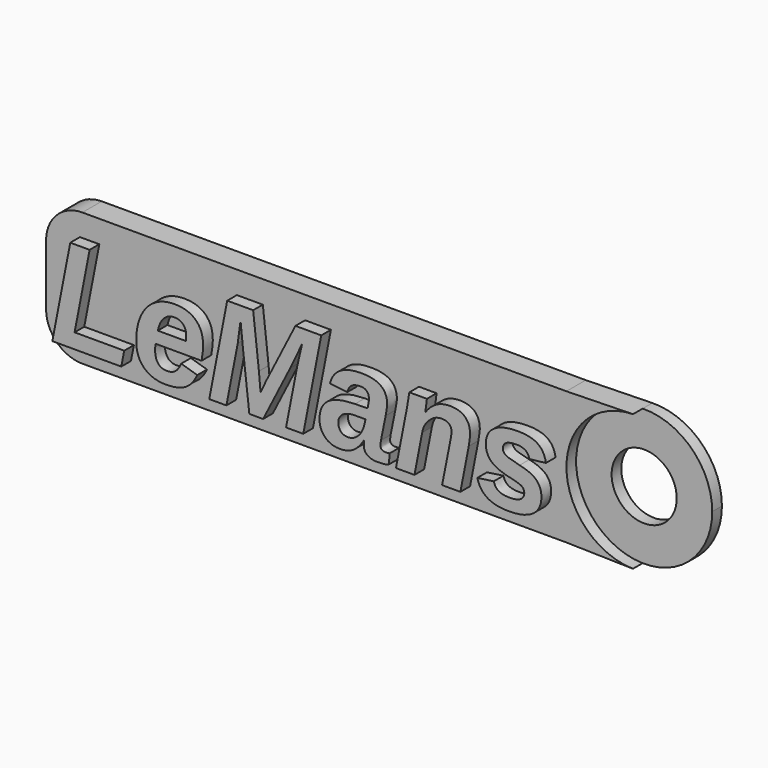
from build123d import *

# Parameters (mm, degrees)
F0_TEXT_SIZE = 11.1111111111
F1_DEPTH     = 1
F2_R         = 2.69
F3_DEPTH     = 2
F4_R         = 3
F5_R         = 5.625
F6_DEPTH     = 1


# Not quite as in the source:
# - Text() gives the source's letters only with a copy of the font that has no kerning and outlines rounded to 1/6400 em; it was checked with that copy


with BuildPart() as f1:
    # F0 (on Front) → F1 (new body)
    with BuildSketch(Plane.XZ):
        with Locations((-20.8784722222, -8)):
            Text('LeMans', F0_TEXT_SIZE, font='Arimo', font_style=FontStyle.BOLDITALIC, text_align=(TextAlign.LEFT, TextAlign.BOTTOM))
    extrude(amount=F1_DEPTH)


with BuildPart() as f3:
    # F2 (on Front) → F3 (new body)
    with BuildSketch(Plane.XZ):
        with BuildLine():
            Line((-22, -9.5), (21, -9.5))
            Line((21, -9.5), (26.4986114618, -9.6235799041))
            ThreePointArc((26.4986114618, -9.6235799041), (21, -4), (26.4986114618, 1.6235799041))
            Line((26.4986114618, 1.6235799041), (21, 1.5))
            Line((21, 1.5), (-22, 1.5))
            Line((-22, 1.5), (-22, -9.5))
        make_face()
        with BuildLine():
            ThreePointArc((26.4986114618, 1.6235799041), (21, -4), (26.4986114618, -9.6235799041))
            ThreePointArc((26.4986114618, -9.6235799041), (30.5575366796, -8.0219125132), (32.25, -4))
            ThreePointArc((32.25, -4), (30.5575366796, 0.0219125132), (26.4986114618, 1.6235799041))
        make_face()
        with Locations((26.625, -4)):
            Circle(F2_R, mode=Mode.SUBTRACT)
    extrude(amount=-F3_DEPTH)

    # F4
    f4_edges = [f3.edges().sort_by_distance(p)[0] for p in [
        (-22, 1, 1.5),
        (-22, 1, -9.5),
        (21, 1, -9.5),
        (21, 1, 1.5),
    ]]
    fillet(f4_edges, radius=F4_R)

    # F5 (on face) → F6 (cut)
    with BuildSketch(Plane.XZ):
        with Locations((26.625, -4)):
            Circle(F5_R)
    extrude(amount=-F6_DEPTH, mode=Mode.SUBTRACT)


solid = Compound([f1.part, f3.part])
